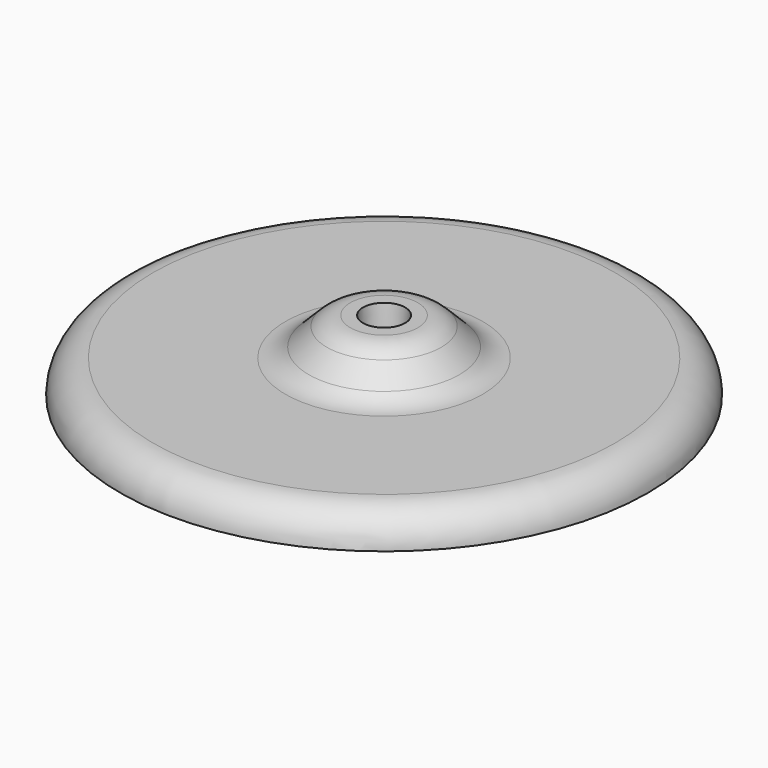
from build123d import *

# Parameters (mm, degrees)
F2_R = 4.99999


# Not quite as in the source:
# - a fillet or chamfer is up to 0.001 mm smaller than in the source, because OpenCascade refuses the exact size


with BuildPart() as f1:
    # F0 (on Front) → F1 (revolve)
    with BuildSketch(Plane.XZ):
        Polygon((40, 5), (12.8825559993, 5), (7.1957559993, 10.6868), (3.1957559993, 10.6868), (2.6416, 2.762), (2.6416, 2), (0, 2), (0, 0), (40, 0), align=None)
    revolve(axis=Axis((0, 0, -11.1281685531), (0, 0, -1)))

    # F2 (radius 5 in the source; OpenCascade refuses exactly that, so slightly less here)
    f2_edges = [f1.edges().sort_by_distance(p)[0] for p in [
        (-12.882556, 0, 5),
        (-40, 0, 5),
        (-7.195756, 0, 10.6868),
    ]]
    fillet(f2_edges, radius=F2_R)


solid = f1.part
